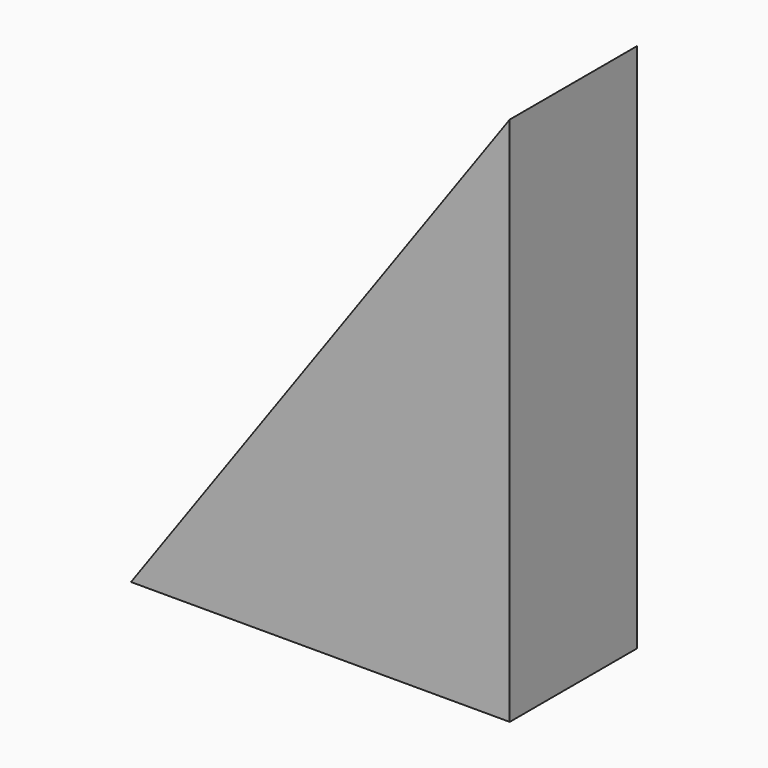
from build123d import *

# Parameters (mm, degrees)
F0_W     = 14.2838
F0_H     = 6
F1_DEPTH = 20
F2_SIZE2 = 19.99999
F2_SIZE  = 14.28379


# Not quite as in the source:
# - a fillet or chamfer is up to 0.001 mm smaller than in the source, because OpenCascade refuses the exact size


with BuildPart() as f1:
    # F0 (on Top) → F1 (new body)
    with BuildSketch(Plane.XY):
        Rectangle(F0_W, F0_H)
    extrude(amount=F1_DEPTH)

    # F2 (size 14.2838 and 20 in the source; OpenCascade refuses exactly that, so slightly less here)
    f2_edges = [f1.edges().sort_by_distance(p)[0] for p in [
        (-7.1419, 0, 20),
    ]]
    f2_side = f1.faces().sort_by_distance((0, 0, 20))[0]
    chamfer(f2_edges, length=F2_SIZE, length2=F2_SIZE2, reference=f2_side)


solid = f1.part
